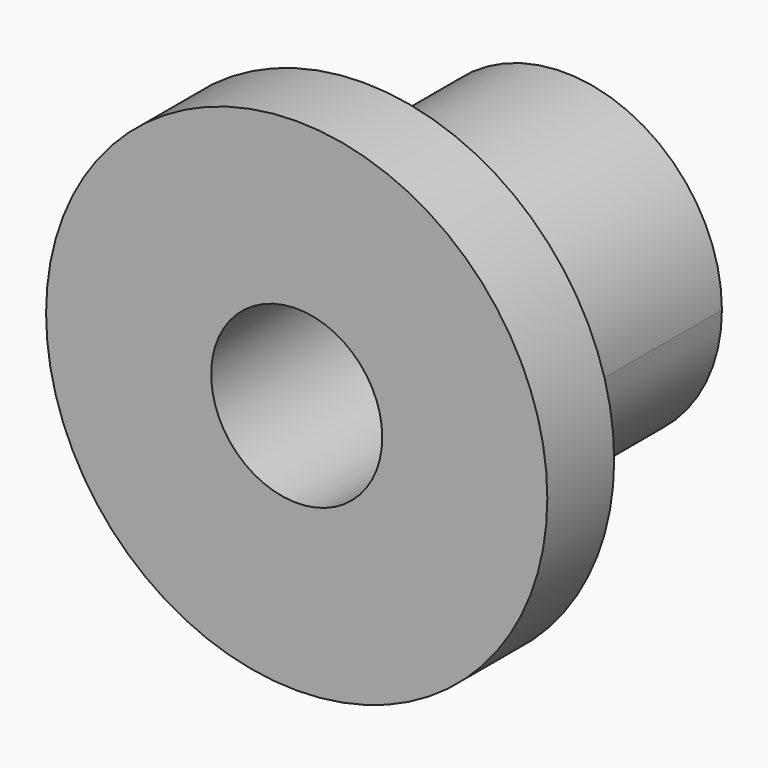
from build123d import *

# Parameters (mm, degrees)
F0_R     = 4.7625
F0_R_2   = 1.6256
F1_DEPTH = 1.5875
F2_DEPTH = 6.35


with BuildPart() as f1:
    # F0 (on Front) → F1 (new body)
    with BuildSketch(Plane.XZ):
        Circle(F0_R)
        with BuildLine():
            ThreePointArc((-1.5702184362, -2.55625), (-1.464469988, 2.6182680639), (3, 0))
            ThreePointArc((3, 0), (2.6182680639, -1.464469988), (1.5702184362, -2.55625))
            ThreePointArc((1.5702184362, -2.55625), (0, -3), (-1.5702184362, -2.55625))
        make_face(mode=Mode.SUBTRACT)
        with BuildLine():
            ThreePointArc((1.5702184362, -2.55625), (2.6182680639, -1.464469988), (3, 0))
            ThreePointArc((3, 0), (-1.464469988, 2.6182680639), (-1.5702184362, -2.55625))
            Line((-1.5702184362, -2.55625), (0, -2.55625))
            Line((0, -2.55625), (1.5702184362, -2.55625))
        make_face()
        Circle(F0_R_2, mode=Mode.SUBTRACT)
        with BuildLine():
            Line((0, -2.55625), (-1.5702184362, -2.55625))
            ThreePointArc((-1.5702184362, -2.55625), (0, -3), (1.5702184362, -2.55625))
            Line((1.5702184362, -2.55625), (0, -2.55625))
        make_face()
    extrude(amount=-F1_DEPTH)

    # F0 (on Front) → F2 (join)
    with BuildSketch(Plane.XZ):
        with BuildLine():
            ThreePointArc((1.5702184362, -2.55625), (2.6182680639, -1.464469988), (3, 0))
            ThreePointArc((3, 0), (-1.464469988, 2.6182680639), (-1.5702184362, -2.55625))
            Line((-1.5702184362, -2.55625), (0, -2.55625))
            Line((0, -2.55625), (1.5702184362, -2.55625))
        make_face()
        Circle(F0_R_2, mode=Mode.SUBTRACT)
    extrude(amount=-F2_DEPTH)


solid = f1.part
